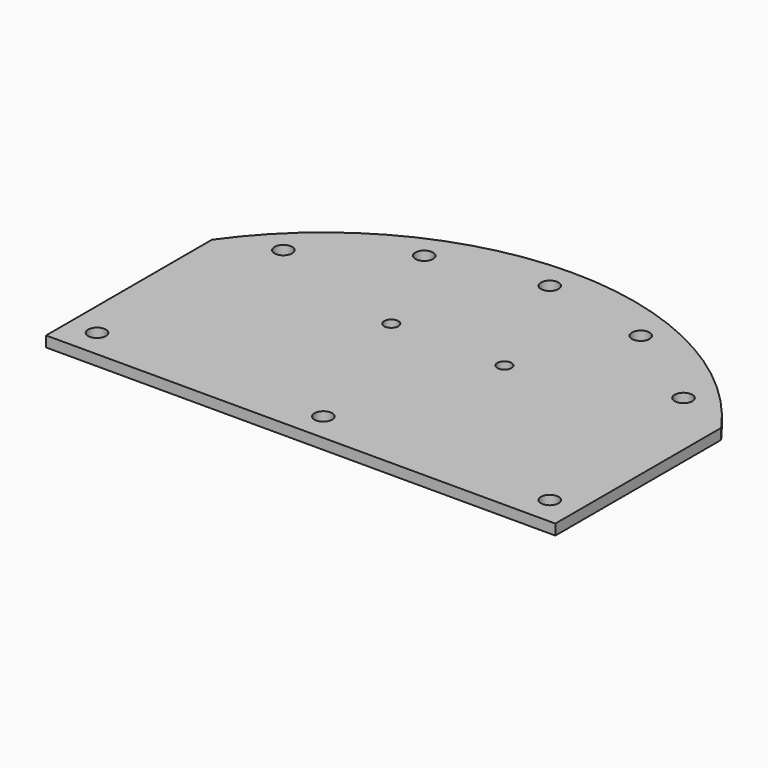
from build123d import *

# Parameters (mm, degrees)
F0_R     = 7.9375
F1_DEPTH = 9.525
F2_W     = 304.8
F2_H     = 50.8
F2_R     = 6.35
F3_DEPTH = 25.4
F4_DEPTH = 9.526


# Not quite as in the source:
# - a feature names something its author has since deleted; it is built from what else it names


with BuildPart() as f1:
    # F0 (on Top) → F1 (new body)
    with BuildSketch(Plane.XY):
        with BuildLine():
            Line((-228.6, 33.6437051366), (-228.6, -152.4))
            Line((-228.6, -152.4), (228.6, -152.4))
            Line((228.6, -152.4), (228.6, 33.6437051366))
            ThreePointArc((228.6, 33.6437051366), (0, 152.4), (-228.6, 33.6437051366))
        make_face()
        with Locations((-203.2, -127)):
            Circle(F0_R, mode=Mode.SUBTRACT)
        with Locations((0, -127)):
            Circle(F0_R, mode=Mode.SUBTRACT)
        with Locations((203.2, -127)):
            Circle(F0_R, mode=Mode.SUBTRACT)
        with Locations((-179.6051224214, 52.6051224214)):
            Circle(F0_R, mode=Mode.SUBTRACT)
        with Locations((-97.2015918207, 107.6654012579)):
            Circle(F0_R, mode=Mode.SUBTRACT)
        with Locations((179.6051224214, 52.6051224214)):
            Circle(F0_R, mode=Mode.SUBTRACT)
        with Locations((97.2015918207, 107.6654012579)):
            Circle(F0_R, mode=Mode.SUBTRACT)
        with Locations((0, 127)):
            Circle(F0_R, mode=Mode.SUBTRACT)
    extrude(amount=-F1_DEPTH)

    # F2 (on face) → F4 (cut, through all)
    with BuildSketch(Plane(origin=(0, 0, -9.525), x_dir=(1, 0, 0), z_dir=(0, 0, -1))):
        with Locations((-50.8, -12.7)):
            Circle(F2_R)
        with Locations((50.8, -12.7)):
            Circle(F2_R)
    extrude(amount=-F4_DEPTH, mode=Mode.SUBTRACT)


with BuildPart() as f3:
    # F2 (on face) → F3 (new body)
    with BuildSketch(Plane(origin=(0, 0, -9.525), x_dir=(1, 0, 0), z_dir=(0, 0, -1))):
        with Locations((0, -12.7)):
            Rectangle(F2_W, F2_H)
        with Locations((-50.8, -12.7)):
            Circle(F2_R, mode=Mode.SUBTRACT)
        with Locations((50.8, -12.7)):
            Circle(F2_R, mode=Mode.SUBTRACT)
    extrude(amount=F3_DEPTH)


solid = Compound([f1.part, f3.part])
